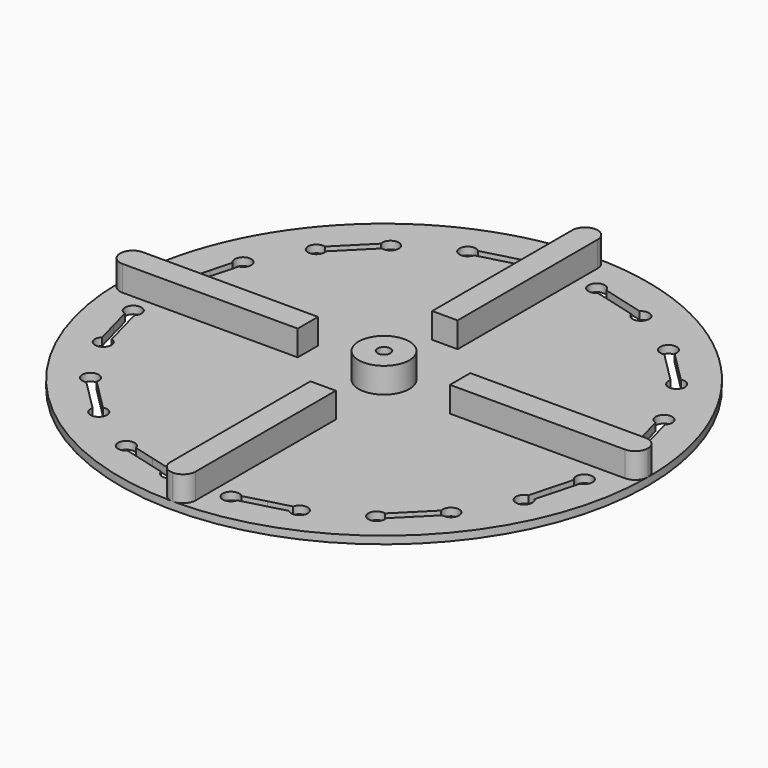
from build123d import *

# Parameters (mm, degrees)
F0_R     = 104
F1_DEPTH = 3
F2_W     = 69
F2_H     = 10
F2_R     = 10
F2_R_2   = 2.55
F3_DEPTH = 10
F4_DEPTH = 3


# Not quite as in the source:
# - a feature names something its author has since deleted; it is built from what else it names


with BuildPart() as f1:
    # F0 (on Top) → F1 (new body)
    with BuildSketch(Plane.XY):
        Circle(F0_R)
    extrude(amount=F1_DEPTH)

    # F2 (on face) → F3 (join)
    with BuildSketch(Plane.XY.offset(3)):
        with Locations((-64.5, 0)):
            Rectangle(F2_W, F2_H)
        with BuildLine():
            ThreePointArc((-104, 0), (-102.5355339059, -3.5355339059), (-99, -5))
            Line((-99, -5), (-99, 5))
            ThreePointArc((-99, 5), (-102.5355339059, 3.5355339059), (-104, 0))
        make_face()
        with BuildLine():
            ThreePointArc((5.0004113768, 98.9999720748), (3.5359525549, 102.5354987085), (0.0004319457, 103.9999720747))
            ThreePointArc((0.0004319457, 103.9999720747), (-3.535115257, 102.5355132529), (-4.9995886232, 98.9999720748))
            Line((-4.9995886232, 98.9999720748), (-4.9995886232, 29.9999720748))
            Line((-4.9995886232, 29.9999720748), (5.0004113768, 29.9999720748))
            Line((5.0004113768, 29.9999720748), (5.0004113768, 98.9999720748))
        make_face()
        with BuildLine():
            ThreePointArc((-5.0026366169, -99.0004113768), (-3.5613838811, -102.5125785011), (-0.0685094531, -103.9999774349))
            ThreePointArc((-0.0685094531, -103.9999774349), (-0.0027697678, -103.9999999631), (0.0629699186, -103.9999809365))
            ThreePointArc((0.0629699186, -103.9999809365), (3.5560171087, -102.5126732778), (4.9973633831, -99.0004113768))
            Line((4.9973633831, -99.0004113768), (4.9973633831, -30.0004113768))
            Line((4.9973633831, -30.0004113768), (-5.0026366169, -30.0004113768))
            Line((-5.0026366169, -30.0004113768), (-5.0026366169, -99.0004113768))
        make_face()
        with BuildLine():
            ThreePointArc((104, 0), (103.9999989259, 0.0149467086), (103.9999957038, 0.0298934169))
            ThreePointArc((103.9999957038, 0.0298934169), (102.523972331, 3.5441133399), (99.0001042186, 4.9969520064))
            Line((99.0001042186, 4.9969520064), (30.0001042186, 4.9969520064))
            Line((30.0001042186, 4.9969520064), (30.0001042186, -5.0030479936))
            Line((30.0001042186, -5.0030479936), (99.0001042186, -5.0030479936))
            ThreePointArc((99.0001042186, -5.0030479936), (102.5238631201, -3.5503178176), (103.9999936659, -0.0362972752))
            ThreePointArc((103.9999936659, -0.0362972752), (103.9999984165, -0.0181486379), (104, 0))
        make_face()
        with Locations((0.0001042186, -2.79252e-05)):
            Circle(F2_R)
        with Locations((0.0001042186, -2.79252e-05)):
            Circle(F2_R_2, mode=Mode.SUBTRACT)
    extrude(amount=F3_DEPTH)

    # F2 (on face) → F4 (cut, through all)
    with BuildSketch(Plane.XY.offset(3)):
        with BuildLine():
            ThreePointArc((-85.513331806, 11.878275299), (-85.7662623092, 13.135285415), (-86.4856853023, 14.196642484))
            ThreePointArc((-86.4856853023, 14.196642484), (-87.9221699094, 15.0175342345), (-89.5766479464, 15.0248634284))
            ThreePointArc((-89.5766479464, 15.0248634284), (-90.7532090061, 9.3086666268), (-85.513331806, 11.878275299))
        make_face()
        with BuildLine():
            Line((-86.4856853023, 14.196642484), (-84.2414314652, 22.5723118292))
            Line((-84.2414314652, 22.5723118292), (-81.9971776281, 30.9479811744))
            ThreePointArc((-81.9971776281, 30.9479811744), (-83.6516556652, 30.9553103683), (-85.0881402722, 31.7762021187))
            Line((-85.0881402722, 31.7762021187), (-87.3323941093, 23.4005327735))
            Line((-87.3323941093, 23.4005327735), (-89.5766479464, 15.0248634284))
            ThreePointArc((-89.5766479464, 15.0248634284), (-87.9221699094, 15.0175342345), (-86.4856853023, 14.196642484))
        make_face()
        with BuildLine():
            ThreePointArc((-85.0881402722, 31.7762021187), (-83.6516556652, 30.9553103683), (-81.9971776281, 30.9479811744))
            ThreePointArc((-81.9971776281, 30.9479811744), (-80.2408850964, 32.1046921035), (-79.5604937686, 34.0945693037))
            ThreePointArc((-79.5604937686, 34.0945693037), (-84.0675038845, 37.0916388005), (-85.0881402722, 31.7762021187))
        make_face()
        with BuildLine():
            ThreePointArc((-67.2625366366, 54.7809925082), (-67.2922516486, 55.2194723778), (-67.3808533111, 55.6499341339))
            ThreePointArc((-67.3808533111, 55.6499341339), (-68.2144395978, 57.079089547), (-69.6435950109, 57.9126758337))
            ThreePointArc((-69.6435950109, 57.9126758337), (-73.0996740782, 52.8139592451), (-67.2625366366, 54.7809925082))
        make_face()
        with BuildLine():
            Line((-67.3808533111, 55.6499341339), (-61.2494378031, 61.7813496419))
            Line((-61.2494378031, 61.7813496419), (-55.118022295, 67.91276515))
            ThreePointArc((-55.118022295, 67.91276515), (-56.5471777082, 68.7463514366), (-57.3807639948, 70.1755068498))
            Line((-57.3807639948, 70.1755068498), (-63.5121795029, 64.0440913417))
            Line((-63.5121795029, 64.0440913417), (-69.6435950109, 57.9126758337))
            ThreePointArc((-69.6435950109, 57.9126758337), (-68.2144395978, 57.079089547), (-67.3808533111, 55.6499341339))
        make_face()
        with BuildLine():
            ThreePointArc((-57.3807639948, 70.1755068498), (-56.5471777082, 68.7463514366), (-55.118022295, 67.91276515))
            ThreePointArc((-55.118022295, 67.91276515), (-52.2820474062, 68.4573110339), (-50.9990806693, 71.0444484755))
            ThreePointArc((-50.9990806693, 71.0444484755), (-54.687560539, 74.2647334635), (-57.3807639948, 70.1755068498))
        make_face()
        with BuildLine():
            ThreePointArc((-30.9371585912, 85.0880844217), (-36.3947847116, 81.9692760214), (-30.1089376468, 81.9971217775))
            ThreePointArc((-30.1089376468, 81.9971217775), (-30.0314823971, 82.4005058629), (-30.0055257762, 82.810437918))
            ThreePointArc((-30.0055257762, 82.810437918), (-30.2474372343, 84.0408457059), (-30.9371585912, 85.0880844217))
        make_face()
        with BuildLine():
            Line((-30.1089376468, 81.9971217775), (-21.7332683017, 84.2413756146))
            Line((-21.7332683017, 84.2413756146), (-13.3575989565, 86.4856294518))
            ThreePointArc((-13.3575989565, 86.4856294518), (-14.1784907069, 87.9221140588), (-14.1858199008, 89.5765920959))
            Line((-14.1858199008, 89.5765920959), (-22.561489246, 87.3323382588))
            Line((-22.561489246, 87.3323382588), (-30.9371585912, 85.0880844217))
            ThreePointArc((-30.9371585912, 85.0880844217), (-30.2474372343, 84.0408457059), (-30.0055257762, 82.810437918))
            ThreePointArc((-30.0055257762, 82.810437918), (-30.0314823971, 82.4005058629), (-30.1089376468, 81.9971217775))
        make_face()
        with BuildLine():
            ThreePointArc((-14.1858199008, 89.5765920959), (-14.1784907069, 87.9221140588), (-13.3575989565, 86.4856294518))
            ThreePointArc((-13.3575989565, 86.4856294518), (-9.8088239837, 85.7551874135), (-7.7892317715, 88.7632759554))
            ThreePointArc((-7.7892317715, 88.7632759554), (-10.6292997163, 91.9873193345), (-14.1858199008, 89.5765920959))
        make_face()
        with BuildLine():
            ThreePointArc((16.1713029323, 89.2694604072), (9.8854558676, 89.2973061633), (15.343081988, 86.1784977631))
            ThreePointArc((15.343081988, 86.1784977631), (16.0328033449, 87.2257364789), (16.274714803, 88.4561442667))
            ThreePointArc((16.274714803, 88.4561442667), (16.2487581821, 88.8660763219), (16.1713029323, 89.2694604072))
        make_face()
        with BuildLine():
            Line((15.343081988, 86.1784977631), (23.7187513332, 83.934243926))
            Line((23.7187513332, 83.934243926), (32.0944206783, 81.6899900889))
            ThreePointArc((32.0944206783, 81.6899900889), (32.1017498722, 83.3444681259), (32.9226416227, 84.780952733))
            Line((32.9226416227, 84.780952733), (24.5469722775, 87.0252065701))
            Line((24.5469722775, 87.0252065701), (16.1713029323, 89.2694604072))
            ThreePointArc((16.1713029323, 89.2694604072), (16.2487581821, 88.8660763219), (16.274714803, 88.4561442667))
            ThreePointArc((16.274714803, 88.4561442667), (16.0328033449, 87.2257364789), (15.343081988, 86.1784977631))
        make_face()
        with BuildLine():
            ThreePointArc((32.9226416227, 84.780952733), (32.1017498722, 83.3444681259), (32.0944206783, 81.6899900889))
            ThreePointArc((32.0944206783, 81.6899900889), (35.6509408628, 79.2792628503), (38.4910088077, 82.5033062293))
            ThreePointArc((38.4910088077, 82.5033062293), (36.4714165955, 85.5113947712), (32.9226416227, 84.780952733))
        make_face()
        with BuildLine():
            ThreePointArc((59.1774320122, 70.2053490974), (53.3402945706, 72.1723823605), (56.7963736378, 67.0736657719))
            ThreePointArc((56.7963736378, 67.0736657719), (58.225529051, 67.9072520585), (59.0591153376, 69.3364074717))
            ThreePointArc((59.0591153376, 69.3364074717), (59.1477170002, 69.7668692277), (59.1774320122, 70.2053490974))
        make_face()
        with BuildLine():
            Line((56.7963736378, 67.0736657719), (62.9277891459, 60.9422502638))
            Line((62.9277891459, 60.9422502638), (69.059204654, 54.8108347558))
            ThreePointArc((69.059204654, 54.8108347558), (69.8927909406, 56.2399901689), (71.3219463538, 57.0735764556))
            Line((71.3219463538, 57.0735764556), (65.1905308457, 63.2049919636))
            Line((65.1905308457, 63.2049919636), (59.0591153376, 69.3364074717))
            ThreePointArc((59.0591153376, 69.3364074717), (58.225529051, 67.9072520585), (56.7963736378, 67.0736657719))
        make_face()
        with BuildLine():
            ThreePointArc((71.3219463538, 57.0735764556), (69.8927909406, 56.2399901689), (69.059204654, 54.8108347558))
            ThreePointArc((69.059204654, 54.8108347558), (71.7524081098, 50.7216081421), (75.4408879794, 53.9418931301))
            ThreePointArc((75.4408879794, 53.9418931301), (74.1579212426, 56.5290305717), (71.3219463538, 57.0735764556))
        make_face()
        with BuildLine():
            ThreePointArc((87.206877422, 32.9483382369), (81.9670002218, 35.5179469091), (83.1435612815, 29.8017501076))
            ThreePointArc((83.1435612815, 29.8017501076), (84.7980393186, 29.8090793015), (86.2345239256, 30.6299710519))
            ThreePointArc((86.2345239256, 30.6299710519), (86.9539469187, 31.6913281209), (87.206877422, 32.9483382369))
        make_face()
        with BuildLine():
            Line((83.1435612815, 29.8017501076), (85.3878151186, 21.4260807624))
            Line((85.3878151186, 21.4260807624), (87.6320689557, 13.0504114172))
            ThreePointArc((87.6320689557, 13.0504114172), (89.0685535628, 13.8713031677), (90.7230315998, 13.8786323616))
            Line((90.7230315998, 13.8786323616), (88.4787777627, 22.2543017067))
            Line((88.4787777627, 22.2543017067), (86.2345239256, 30.6299710519))
            ThreePointArc((86.2345239256, 30.6299710519), (84.7980393186, 29.8090793015), (83.1435612815, 29.8017501076))
        make_face()
        with BuildLine():
            ThreePointArc((90.7230315998, 13.8786323616), (89.0685535628, 13.8713031677), (87.6320689557, 13.0504114172))
            ThreePointArc((87.6320689557, 13.0504114172), (88.6527053434, 7.7349747355), (93.1597154593, 10.7320442322))
            ThreePointArc((93.1597154593, 10.7320442322), (92.4793241316, 12.7219214324), (90.7230315998, 13.8786323616))
        make_face()
        with BuildLine():
            ThreePointArc((92.8525837707, -13.3319023423), (88.3455736547, -10.3348328455), (87.324937267, -15.6502695273))
            ThreePointArc((87.324937267, -15.6502695273), (88.7614218741, -16.4711612777), (90.4158999111, -16.4784904716))
            ThreePointArc((90.4158999111, -16.4784904716), (92.1721924429, -15.3217795424), (92.8525837707, -13.3319023423))
        make_face()
        with BuildLine():
            Line((87.324937267, -15.6502695273), (85.0806834299, -24.0259388724))
            Line((85.0806834299, -24.0259388724), (82.8364295928, -32.4016082176))
            ThreePointArc((82.8364295928, -32.4016082176), (84.4909076299, -32.4089374115), (85.9273922369, -33.2298291619))
            Line((85.9273922369, -33.2298291619), (88.171646074, -24.8541598168))
            Line((88.171646074, -24.8541598168), (90.4158999111, -16.4784904716))
            ThreePointArc((90.4158999111, -16.4784904716), (88.7614218741, -16.4711612777), (87.324937267, -15.6502695273))
        make_face()
        with BuildLine():
            ThreePointArc((85.9273922369, -33.2298291619), (84.4909076299, -32.4089374115), (82.8364295928, -32.4016082176))
            ThreePointArc((82.8364295928, -32.4016082176), (81.6598685331, -38.1178050191), (86.8997457333, -35.5481963469))
            ThreePointArc((86.8997457333, -35.5481963469), (86.6468152301, -34.291186231), (85.9273922369, -33.2298291619))
        make_face()
        with BuildLine():
            ThreePointArc((74.6017886013, -56.2346195514), (70.9133087317, -53.0143345634), (68.2201052758, -57.1035611771))
            ThreePointArc((68.2201052758, -57.1035611771), (69.0536915625, -58.5327165903), (70.4828469756, -59.3663028769))
            ThreePointArc((70.4828469756, -59.3663028769), (73.3188218645, -58.821756993), (74.6017886013, -56.2346195514))
        make_face()
        with BuildLine():
            Line((68.2201052758, -57.1035611771), (62.0886897678, -63.2349766852))
            Line((62.0886897678, -63.2349766852), (55.9572742597, -69.3663921932))
            ThreePointArc((55.9572742597, -69.3663921932), (57.3864296729, -70.1999784798), (58.2200159595, -71.629133893))
            Line((58.2200159595, -71.629133893), (64.3514314676, -65.497718385))
            Line((64.3514314676, -65.497718385), (70.4828469756, -59.3663028769))
            ThreePointArc((70.4828469756, -59.3663028769), (69.0536915625, -58.5327165903), (68.2201052758, -57.1035611771))
        make_face()
        with BuildLine():
            ThreePointArc((58.2200159595, -71.629133893), (57.3864296729, -70.1999784798), (55.9572742597, -69.3663921932))
            ThreePointArc((55.9572742597, -69.3663921932), (52.5011951924, -74.4651087818), (58.338332634, -72.4980755187))
            ThreePointArc((58.338332634, -72.4980755187), (58.308617622, -72.0595956491), (58.2200159595, -71.629133893))
        make_face()
        with BuildLine():
            ThreePointArc((37.3447777409, -84.2640649612), (34.504709796, -81.0400215822), (30.9481896115, -83.4507488208))
            ThreePointArc((30.9481896115, -83.4507488208), (30.9555188054, -85.1052268578), (31.7764105559, -86.5417114649))
            ThreePointArc((31.7764105559, -86.5417114649), (35.3251855287, -87.2721535031), (37.3447777409, -84.2640649612))
        make_face()
        with BuildLine():
            Line((30.9481896115, -83.4507488208), (22.5725202664, -85.6950026579))
            Line((22.5725202664, -85.6950026579), (14.1968509212, -87.939256495))
            ThreePointArc((14.1968509212, -87.939256495), (14.8865722781, -88.9864952108), (15.1284837362, -90.2169029986))
            ThreePointArc((15.1284837362, -90.2169029986), (15.1025271153, -90.6268350538), (15.0250718655, -91.0302191391))
            Line((15.0250718655, -91.0302191391), (23.4007412107, -88.785965302))
            Line((23.4007412107, -88.785965302), (31.7764105559, -86.5417114649))
            ThreePointArc((31.7764105559, -86.5417114649), (30.9555188054, -85.1052268578), (30.9481896115, -83.4507488208))
        make_face()
        with BuildLine():
            ThreePointArc((15.1284837362, -90.2169029986), (14.8865722781, -88.9864952108), (14.1968509212, -87.939256495))
            ThreePointArc((14.1968509212, -87.939256495), (8.7392248008, -91.0580648952), (15.0250718655, -91.0302191391))
            ThreePointArc((15.0250718655, -91.0302191391), (15.1025271153, -90.6268350538), (15.1284837362, -90.2169029986))
        make_face()
        with BuildLine():
            ThreePointArc((-8.9354628383, -89.9097713099), (-10.9550550505, -86.9016827681), (-14.5038300233, -87.6321248063))
            ThreePointArc((-14.5038300233, -87.6321248063), (-15.3247217737, -89.0686094133), (-15.3320509676, -90.7230874504))
            ThreePointArc((-15.3320509676, -90.7230874504), (-11.7755307831, -93.133814689), (-8.9354628383, -89.9097713099))
        make_face()
        with BuildLine():
            ThreePointArc((-31.2551687136, -83.1436171321), (-31.1777134639, -83.5470012174), (-31.151756843, -83.9569332726))
            ThreePointArc((-31.151756843, -83.9569332726), (-31.3936683011, -85.1873410604), (-32.083389658, -86.2345797762))
            Line((-32.083389658, -86.2345797762), (-23.7077203128, -88.4788336133))
            Line((-23.7077203128, -88.4788336133), (-15.3320509676, -90.7230874504))
            ThreePointArc((-15.3320509676, -90.7230874504), (-15.3247217737, -89.0686094133), (-14.5038300233, -87.6321248063))
            Line((-14.5038300233, -87.6321248063), (-22.8794993685, -85.3878709692))
            Line((-22.8794993685, -85.3878709692), (-31.2551687136, -83.1436171321))
        make_face()
        with BuildLine():
            ThreePointArc((-32.083389658, -86.2345797762), (-31.3936683011, -85.1873410604), (-31.151756843, -83.9569332726))
            ThreePointArc((-31.151756843, -83.9569332726), (-31.1777134639, -83.5470012174), (-31.2551687136, -83.1436171321))
            ThreePointArc((-31.2551687136, -83.1436171321), (-37.5410157784, -83.115771376), (-32.083389658, -86.2345797762))
        make_face()
        with BuildLine():
            ThreePointArc((-51.8381800475, -71.6589761406), (-53.1211467843, -69.071838699), (-55.9571216731, -68.5272928151))
            ThreePointArc((-55.9571216731, -68.5272928151), (-57.3862770863, -69.3608791017), (-58.2198633729, -70.7900345149))
            ThreePointArc((-58.2198633729, -70.7900345149), (-55.5266599171, -74.8792611286), (-51.8381800475, -71.6589761406))
        make_face()
        with BuildLine():
            Line((-55.9571216731, -68.5272928151), (-62.0885371812, -62.395877307))
            Line((-62.0885371812, -62.395877307), (-68.2199526893, -56.264461799))
            ThreePointArc((-68.2199526893, -56.264461799), (-69.0535389759, -57.6936172122), (-70.482694389, -58.5272034988))
            Line((-70.482694389, -58.5272034988), (-64.351278881, -64.6586190068))
            Line((-64.351278881, -64.6586190068), (-58.2198633729, -70.7900345149))
            ThreePointArc((-58.2198633729, -70.7900345149), (-57.3862770863, -69.3608791017), (-55.9571216731, -68.5272928151))
        make_face()
        with BuildLine():
            ThreePointArc((-70.482694389, -58.5272034988), (-69.0535389759, -57.6936172122), (-68.2199526893, -56.264461799))
            ThreePointArc((-68.2199526893, -56.264461799), (-68.1313510267, -55.8340000429), (-68.1016360147, -55.3955201733))
            ThreePointArc((-68.1016360147, -55.3955201733), (-73.9387734563, -53.4284869102), (-70.482694389, -58.5272034988))
        make_face()
        with BuildLine():
            ThreePointArc((-79.8676254573, -34.4019652801), (-80.5480167851, -32.41208808), (-82.3043093168, -31.2553771508))
            ThreePointArc((-82.3043093168, -31.2553771508), (-83.9587873539, -31.2627063447), (-85.3952719609, -32.0835980951))
            ThreePointArc((-85.3952719609, -32.0835980951), (-84.3746355732, -37.3990347769), (-79.8676254573, -34.4019652801))
        make_face()
        with BuildLine():
            Line((-82.3043093168, -31.2553771508), (-84.5485631539, -22.8797078056))
            Line((-84.5485631539, -22.8797078056), (-86.792816991, -14.5040384605))
            ThreePointArc((-86.792816991, -14.5040384605), (-88.2293015981, -15.3249302109), (-89.8837796351, -15.3322594048))
            Line((-89.8837796351, -15.3322594048), (-87.639525798, -23.70792875))
            Line((-87.639525798, -23.70792875), (-85.3952719609, -32.0835980951))
            ThreePointArc((-85.3952719609, -32.0835980951), (-83.9587873539, -31.2627063447), (-82.3043093168, -31.2553771508))
        make_face()
        with BuildLine():
            ThreePointArc((-89.8837796351, -15.3322594048), (-88.2293015981, -15.3249302109), (-86.792816991, -14.5040384605))
            ThreePointArc((-86.792816991, -14.5040384605), (-86.0733939979, -13.4426813914), (-85.8204634946, -12.1856712755))
            ThreePointArc((-85.8204634946, -12.1856712755), (-91.0603406948, -9.6160626033), (-89.8837796351, -15.3322594048))
        make_face()
        with Locations((0.0001042186, -2.79252e-05)):
            Circle(F2_R_2)
    extrude(amount=-F4_DEPTH, mode=Mode.SUBTRACT)


solid = f1.part
